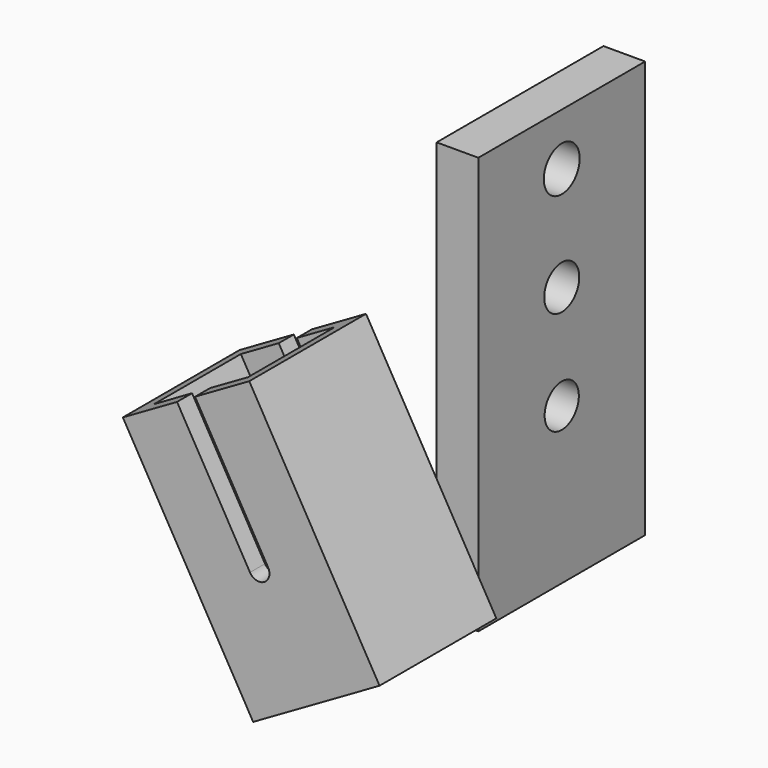
from build123d import *

# Parameters (mm, degrees)
F0_W     = 1.8
F0_H     = 2
F1_DEPTH = 25
F0_W_2   = 20
F0_H_2   = 40
F0_R     = 2.05
F0_R_2   = 2.1
F0_R_3   = 2.15
F2_DEPTH = 4
F3_DEPTH = 15
F4_ANGLE = -60
F6_R     = 0.99999


# Not quite as in the source:
# - a fillet or chamfer is up to 0.001 mm smaller than in the source, because OpenCascade refuses the exact size


with BuildPart() as f1:
    # F0 (on Right) → F1 (new body)
    with BuildSketch(Plane.YZ):
        Polygon((7, 8), (7, 14), (-7, 14), (-7, 8), (-5.2, 8), (-5.2, 12.2), (5.2, 12.2), (5.2, 8), align=None)
        Polygon((7, 0), (7, 6), (5.2, 6), (5.2, 1.8), (-5.2, 1.8), (-5.2, 6), (-7, 6), (-7, 0), align=None)
        with Locations((6.1, 7)):
            Rectangle(F0_W, F0_H)
        Polygon((5.2, 6), (5.2, 8), (5.2, 12.2), (-5.2, 12.2), (-5.2, 8), (-5.2, 6), (-5.2, 1.8), (5.2, 1.8), align=None)
        with Locations((-6.1, 7)):
            Rectangle(F0_W, F0_H)
    extrude(amount=F1_DEPTH)

    # F0 (on Right) → F3 (cut)
    with BuildSketch(Plane.YZ):
        Polygon((5.2, 6), (5.2, 8), (5.2, 12.2), (-5.2, 12.2), (-5.2, 8), (-5.2, 6), (-5.2, 1.8), (5.2, 1.8), align=None)
        with Locations((6.1, 7)):
            Rectangle(F0_W, F0_H)
        with Locations((-6.1, 7)):
            Rectangle(F0_W, F0_H)
    extrude(amount=F3_DEPTH, mode=Mode.SUBTRACT)


with BuildPart() as f2:
    # F0 (on Right) → F2 (new body)
    with BuildSketch(Plane.YZ):
        with Locations((25, 20)):
            Rectangle(F0_W_2, F0_H_2)
        with Locations((25, 15)):
            Circle(F0_R, mode=Mode.SUBTRACT)
        with Locations((25, 25)):
            Circle(F0_R_2, mode=Mode.SUBTRACT)
        with Locations((25, 35)):
            Circle(F0_R_3, mode=Mode.SUBTRACT)
    extrude(amount=F2_DEPTH)


with BuildPart() as f1_1:
    # F4: moved
    add(f1.part.rotate(Axis((25, 0, 0), (0, -1, 0)), F4_ANGLE))


with BuildPart() as f1_2:
    # F5: moved
    add(f1_1.part.moved(Location((-25, 0, 0))))

    # F6 (radius 1 in the source; OpenCascade refuses exactly that, so slightly less here)
    f6_edges = [f1_2.edges().sort_by_distance(p)[0] for p in [
        (1.928203, -6.1, 12.660254),
        (0.196152, -6.1, 11.660254),
        (1.928203, 6.1, 12.660254),
        (0.196152, 6.1, 11.660254),
    ]]
    fillet(f6_edges, radius=F6_R)


solid = Compound([f2.part, f1_2.part])
